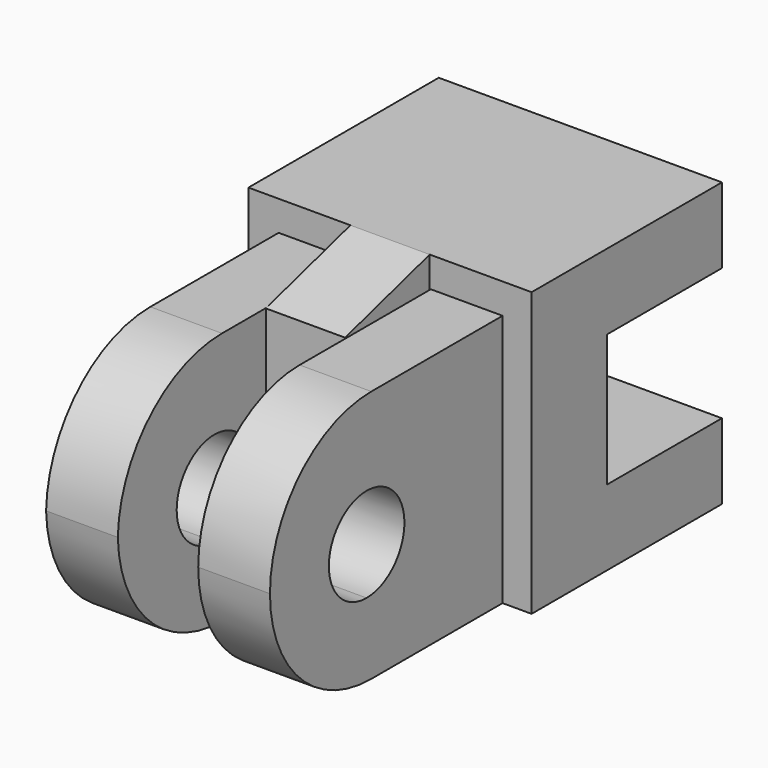
from build123d import *

# Parameters (mm, degrees)
F1_DEPTH     = 75
F2_W         = 21
F2_H         = 75
F3_DEPTH     = 28
F5_DEPTH     = 50.8
F6_W         = 19
F6_H         = 77
F7_DEPTH     = 75
F9_DEPTH     = 38.6
F11_DEPTH    = 19
F12_W        = 19
F12_H        = 77
F13_DEPTH    = 77
F14_W        = 19
F14_H        = 9.9398646951
F15_DEPTH    = 77
F17_DEPTH    = 75.4
F18_T1_DEPTH = 19
F19_T1_DEPTH = 102.8939212925
F19_T3_DEPTH = 186.7878425849


# Not quite as in the source:
# - a fillet or chamfer that OpenCascade refuses, or shapes differently, is made with other operations: its cross-section is extruded or revolved along the edge and cut away or added


with BuildPart() as f1:
    # F0 (on Right) → F1 (new body)
    with BuildSketch(Plane.YZ):
        Polygon((0, 75), (0, 0), (63, 0), (63, 20), (25, 20), (25, 55), (63, 55), (63, 75), align=None)
    extrude(amount=F1_DEPTH)

    # F2 (on face) → F3 (join)
    with BuildSketch(Plane.XZ):
        with Locations((37.5, 37.5)):
            Rectangle(F2_W, F2_H)
    extrude(amount=F3_DEPTH)

    # F4 (on face) → F5 (cut)
    with BuildSketch(Plane(origin=(27, 0, 0), x_dir=(0, -1, 0), z_dir=(-1, 0, 0))):
        Polygon((28, 67), (28, 75), (0, 75), align=None)
    extrude(amount=-F5_DEPTH, mode=Mode.SUBTRACT)

    # F6 (on Top) → F7 (join)
    with BuildSketch(Plane.XY):
        with Locations((57.8057536185, -38.5)):
            Rectangle(F6_W, F6_H)
    extrude(amount=F7_DEPTH)

    # F8 (on face) → F9 (cut)
    with BuildSketch(Plane(origin=(48.3057536185, 0, 0), x_dir=(0, -1, 0), z_dir=(-1, 0, 0))):
        Polygon((77, 75), (0, 75), (27.784453705, 67), (77, 67), align=None)
    extrude(amount=-F9_DEPTH, mode=Mode.SUBTRACT)

    # F10 (on face) → F11 (cut)
    with BuildSketch(Plane.YZ.offset(67.3057536185)):
        Polygon((0, 75), (-27.784453705, 67), (0, 67), align=None)
    extrude(amount=-F11_DEPTH, mode=Mode.SUBTRACT)

    # F12 (on Top) → F13 (join)
    with BuildSketch(Plane.XY):
        with Locations((17.5, -38.5)):
            Rectangle(F12_W, F12_H)
    extrude(amount=F13_DEPTH)

    # F14 (on face) → F15 (cut)
    with BuildSketch(Plane.XZ.offset(77)):
        with Locations((17.5, 72.0300676525)):
            Rectangle(F14_W, F14_H)
    extrude(amount=-F15_DEPTH, mode=Mode.SUBTRACT)

    # F16 (on face) → F17 (cut)
    with BuildSketch(Plane(origin=(8, 0, 0), x_dir=(0, -1, 0), z_dir=(-1, 0, 0))):
        with BuildLine():
            ThreePointArc((57.5, 32), (36.1611652352, 40.8388347648), (45, 19.5))
            ThreePointArc((45, 19.5), (53.8388347648, 23.1611652352), (57.5, 32))
        make_face()
    extrude(amount=-F17_DEPTH, mode=Mode.SUBTRACT)

    # F18: fillet of radius 34.5232539419 on 2 edges, made by hand

    # F18_s2 → F18_t1 (cut)
    with BuildSketch(Plane.YZ.offset(8)):
        with BuildLine():
            ThreePointArc((-42.4767460581, 67.0601353049), (-66.888373029, 56.948508334), (-77, 32.536881363))
            Line((-77, 32.536881363), (-77.6904650788, 32.536881363))
            Line((-77.6904650788, 32.536881363), (-77.6904650788, 67.7506003838))
            Line((-77.6904650788, 67.7506003838), (-42.4767460581, 67.7506003838))
            Line((-42.4767460581, 67.7506003838), (-42.4767460581, 67.0601353049))
        make_face()
        with BuildLine():
            ThreePointArc((-42.4767460581, 0), (-66.888373029, 10.111626971), (-77, 34.5232539419))
            Line((-77, 34.5232539419), (-77.6904650788, 34.5232539419))
            Line((-77.6904650788, 34.5232539419), (-77.6904650788, -0.6904650788))
            Line((-77.6904650788, -0.6904650788), (-42.4767460581, -0.6904650788))
            Line((-42.4767460581, -0.6904650788), (-42.4767460581, 0))
        make_face()
    extrude(amount=F18_T1_DEPTH, mode=Mode.SUBTRACT)

    # F19: fillet of radius 33.557568517 on 2 edges, made by hand

    # F19_s2 → F19_t1 (cut)
    with BuildSketch(Plane.YZ.offset(48.3057536185)):
        with BuildLine():
            ThreePointArc((-77, 33.442431483), (-67.1712157415, 57.1712157415), (-43.442431483, 67))
            Line((-43.442431483, 67), (-77, 67))
            Line((-77, 67), (-77, 33.442431483))
        make_face()
    extrude(amount=F19_T1_DEPTH, mode=Mode.SUBTRACT)

    # F19_s4 → F19_t3 (cut)
    with BuildSketch(Plane.YZ.offset(-35.588167674)):
        with BuildLine():
            ThreePointArc((-43.442431483, 0), (-67.1712157415, 9.8287842585), (-77, 33.557568517))
            Line((-77, 33.557568517), (-77, 0))
            Line((-77, 0), (-43.442431483, 0))
        make_face()
    extrude(amount=F19_T3_DEPTH, mode=Mode.SUBTRACT)


solid = f1.part
